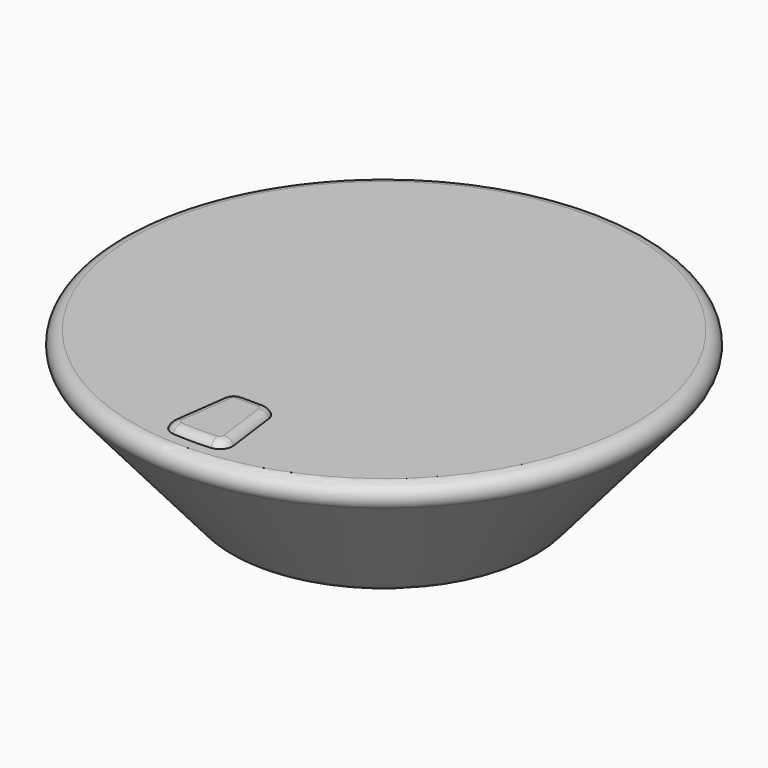
from build123d import *

# Parameters (mm, degrees)
F3_DEPTH     = 3.175
F4_T1_DEPTH  = 26.7171757075
F4_T3_DEPTH  = 10.7537660931
F4_T5_DEPTH  = 26.7171757075
F4_T8_ANGLE  = 93.1775029202
F4_T10_ANGLE = 82.3499629572
F4_T12_ANGLE = 82.3499629572
F4_T14_ANGLE = 93.1775029202
F4_T16_ANGLE = 8.9450682453


# Not quite as in the source:
# - a fillet or chamfer that OpenCascade refuses, or shapes differently, is made with other operations: its cross-section is extruded or revolved along the edge and cut away or added


with BuildPart() as f1:
    # F0 (on Front) → F1 (revolve)
    with BuildSketch(Plane.XZ):
        with BuildLine():
            Line((126.2178106584, 0), (0, 0))
            Line((0, 0), (0, -75.8794099092))
            Line((0, -75.8794099092), (72.1120906848, -75.8794099092))
            ThreePointArc((72.1120906848, -75.8794099092), (74.7667467473, -75.2978846808), (76.9351825033, -73.6598197328))
            Line((76.9351825033, -73.6598197328), (131.0409024769, -10.4804098236))
            ThreePointArc((131.0409024769, -10.4804098236), (131.98628543, -3.6953439375), (126.2178106584, 0))
        make_face()
    revolve(axis=Axis((0, 0, -37.9397049546), (0, 0, -1)))

    # F2 (on face) → F3 (join)
    with BuildSketch(Plane.XY):
        with BuildLine():
            Line((15.2270092071, -113.3658299561), (11.6703658958, -86.8864461614))
            ThreePointArc((11.6703658958, -86.8864461614), (9.5574744515, -82.9521101243), (5.3768830466, -81.3817707299))
            Line((5.3768830466, -81.3817707299), (0, -81.3817707299))
            Line((0, -81.3817707299), (-5.3768830466, -81.3817707299))
            ThreePointArc((-5.3768830466, -81.3817707299), (-9.5574744515, -82.9521101243), (-11.6703658958, -86.8864461614))
            Line((-11.6703658958, -86.8864461614), (-15.2270092071, -113.3658299561))
            ThreePointArc((-15.2270092071, -113.3658299561), (-13.8726748488, -118.2020582047), (-9.4287069428, -120.5418176958))
            ThreePointArc((-9.4287069428, -120.5418176958), (0, -120.9100092136), (9.4287069428, -120.5418176958))
            ThreePointArc((9.4287069428, -120.5418176958), (13.8726748488, -118.2020582047), (15.2270092071, -113.3658299561))
        make_face()
    extrude(amount=F3_DEPTH)

    # F4: fillet of radius 5.08 on 1 edges, made by hand

    # F4_s2 → F4_t1 (cut)
    with BuildSketch(Plane(origin=(15.2270092071, -113.3658299561, 0), x_dir=(0, 0, 1), z_dir=(-0.1331219793, 0.9910996613, 0))):
        with BuildLine():
            ThreePointArc((0, 0), (2.3071134838, -1.8694797079), (3.175, -4.7092860393))
            Line((3.175, -4.7092860393), (3.175, 0))
            Line((3.175, 0), (0, 0))
        make_face()
    extrude(amount=F4_T1_DEPTH, mode=Mode.SUBTRACT)

    # F4_s4 → F4_t3 (cut)
    with BuildSketch(Plane.YZ.offset(-5.3768830466)):
        with BuildLine():
            ThreePointArc((-81.3817707299, 0), (-83.2512504378, 2.3071134838), (-86.0910567692, 3.175))
            Line((-86.0910567692, 3.175), (-81.3817707299, 3.175))
            Line((-81.3817707299, 3.175), (-81.3817707299, 0))
        make_face()
    extrude(amount=F4_T3_DEPTH, mode=Mode.SUBTRACT)

    # F4_s6 → F4_t5 (cut)
    with BuildSketch(Plane(origin=(-11.6703658958, -86.8864461614, 0), x_dir=(0, 0, 1), z_dir=(-0.1331219793, -0.9910996613, 0))):
        with BuildLine():
            ThreePointArc((0, 0), (2.3071134838, -1.8694797079), (3.175, -4.7092860393))
            Line((3.175, -4.7092860393), (3.175, 0))
            Line((3.175, 0), (0, 0))
        make_face()
    extrude(amount=F4_T5_DEPTH, mode=Mode.SUBTRACT)

    # F4_s7 → F4_t8 (revolve, cut)
    with BuildSketch(Plane(origin=(0, 0, 0), x_dir=(0, 0, 1), z_dir=(-0.9969548301, -0.0779811945, 0))):
        with BuildLine():
            ThreePointArc((0, -120.9100092136), (2.3071134838, -119.0405295057), (3.175, -116.2007231743))
            Line((3.175, -116.2007231743), (3.175, -120.9100092136))
            Line((3.175, -120.9100092136), (0, -120.9100092136))
        make_face()
    revolve(axis=Axis((8.9335263578, -114.2111545246, 3.175), (0, 0, 1)), revolution_arc=F4_T8_ANGLE, mode=Mode.SUBTRACT)

    # F4_s9 → F4_t10 (revolve, cut)
    with BuildSketch(Plane(origin=(11.6703658958, -86.8864461614, 0), x_dir=(0, 0, 1), z_dir=(0.1331219793, -0.9910996613, 0))):
        with BuildLine():
            ThreePointArc((0, 0), (2.3071134838, 1.8694797079), (3.175, 4.7092860393))
            Line((3.175, 4.7092860393), (3.175, 0))
            Line((3.175, 0), (0, 0))
        make_face()
    revolve(axis=Axis((5.3768830466, -87.7317707299, 3.175), (0, 0, 1)), revolution_arc=F4_T10_ANGLE, mode=Mode.SUBTRACT)

    # F4_s11 → F4_t12 (revolve, cut)
    with BuildSketch(Plane.YZ.offset(-5.3768830466)):
        with BuildLine():
            ThreePointArc((-81.3817707299, 0), (-83.2512504378, 2.3071134838), (-86.0910567692, 3.175))
            Line((-86.0910567692, 3.175), (-81.3817707299, 3.175))
            Line((-81.3817707299, 3.175), (-81.3817707299, 0))
        make_face()
    revolve(axis=Axis((-5.3768830466, -87.7317707299, 3.175), (0, 0, 1)), revolution_arc=F4_T12_ANGLE, mode=Mode.SUBTRACT)

    # F4_s13 → F4_t14 (revolve, cut)
    with BuildSketch(Plane(origin=(-15.2270092071, -113.3658299561, 0), x_dir=(0, 0, 1), z_dir=(0.1331219793, 0.9910996613, 0))):
        with BuildLine():
            ThreePointArc((0, 0), (2.3071134838, 1.8694797079), (3.175, 4.7092860393))
            Line((3.175, 4.7092860393), (3.175, 0))
            Line((3.175, 0), (0, 0))
        make_face()
    revolve(axis=Axis((-8.9335263578, -114.2111545246, 3.175), (0, 0, 1)), revolution_arc=F4_T14_ANGLE, mode=Mode.SUBTRACT)

    # F4_s15 → F4_t16 (revolve, cut)
    with BuildSketch(Plane(origin=(0, 0, 0), x_dir=(0, 0, 1), z_dir=(-0.9969548301, 0.0779811945, 0))):
        with BuildLine():
            ThreePointArc((0, -120.9100092136), (2.3071134838, -119.0405295057), (3.175, -116.2007231743))
            Line((3.175, -116.2007231743), (3.175, -120.9100092136))
            Line((3.175, -120.9100092136), (0, -120.9100092136))
        make_face()
    revolve(axis=Axis((0, 0, 3.175), (0, 0, 1)), revolution_arc=F4_T16_ANGLE, mode=Mode.SUBTRACT)


solid = f1.part
